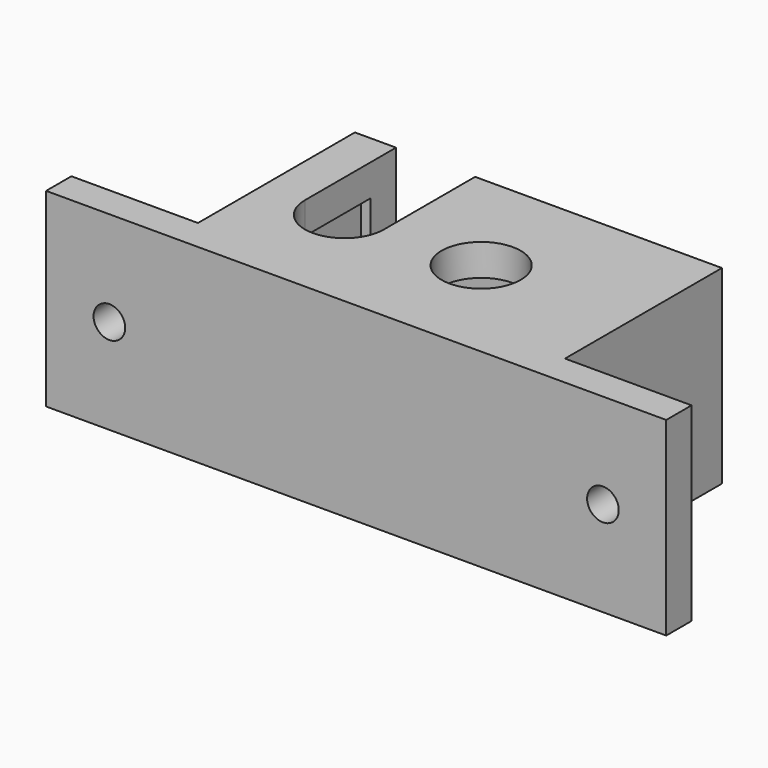
from build123d import *

# Parameters (mm, degrees)
F1_DEPTH = 30
F0_R     = 6.25
F2_DEPTH = 5
F3_W     = 5
F3_H     = 30
F4_DEPTH = 20
F5_W     = 5
F5_H     = 30
F6_DEPTH = 20
F7_R     = 2.5
F8_DEPTH = 25


# Not quite as in the source:
# - a feature names something its author has since deleted; it is built from what else it names


with BuildPart() as f1:
    # F0 (on Top) → F1 (new body)
    with BuildSketch(Plane.XY):
        Polygon((25.3224579843, 32.3690634753), (25.3224579843, 6.3690634753), (30.3224579843, 6.3690634753), (30.3224579843, 37.3690634753), (-8.6790506474, 37.3690634753), (-8.6790506474, 32.3690634753), align=None)
        Polygon((-22.6775420157, 6.3690634753), (-22.6775420157, 32.3690634753), (-21.1775420157, 32.3690634753), (-21.1775420157, 37.3690634753), (-27.6775420157, 37.3690634753), (-27.6775420157, 6.3690634753), align=None)
        Polygon((25.3224579843, 6.3690634753), (-22.6775420157, 6.3690634753), (-27.6775420157, 6.3690634753), (-27.6775420157, 1.3690634753), (30.3224579843, 1.3690634753), (30.3224579843, 6.3690634753), align=None)
    extrude(amount=-F1_DEPTH)

    # F0 (on Top) → F2 (join)
    with BuildSketch(Plane.XY):
        Polygon((-22.6775420157, 6.3690634753), (-22.6775420157, 32.3690634753), (-21.1775420157, 32.3690634753), (-21.1775420157, 37.3690634753), (-27.6775420157, 37.3690634753), (-27.6775420157, 6.3690634753), align=None)
        with BuildLine():
            Line((-21.1775420157, 32.3690634753), (-22.6775420157, 32.3690634753))
            Line((-22.6775420157, 32.3690634753), (-22.6775420157, 6.3690634753))
            Line((-22.6775420157, 6.3690634753), (25.3224579843, 6.3690634753))
            Line((25.3224579843, 6.3690634753), (25.3224579843, 32.3690634753))
            Line((25.3224579843, 32.3690634753), (-8.6790506474, 32.3690634753))
            Line((-8.6790506474, 32.3690634753), (-8.6790506474, 19.5063792474))
            ThreePointArc((-8.6790506474, 19.5063792474), (-14.858879986, 13.1194406446), (-21.1775420157, 19.3690634753))
            Line((-21.1775420157, 19.3690634753), (-21.1775420157, 32.3690634753))
        make_face()
        with Locations((6.6724579843, 19.3690634753)):
            Circle(F0_R, mode=Mode.SUBTRACT)
        Polygon((25.3224579843, 6.3690634753), (-22.6775420157, 6.3690634753), (-27.6775420157, 6.3690634753), (-27.6775420157, 1.3690634753), (30.3224579843, 1.3690634753), (30.3224579843, 6.3690634753), align=None)
        Polygon((25.3224579843, 32.3690634753), (25.3224579843, 6.3690634753), (30.3224579843, 6.3690634753), (30.3224579843, 37.3690634753), (-8.6790506474, 37.3690634753), (-8.6790506474, 32.3690634753), align=None)
    extrude(amount=-F2_DEPTH)

    # F3 (on face) → F4 (join)
    with BuildSketch(Plane.YZ.offset(30.3224579843)):
        with Locations((3.8690634753, -15)):
            Rectangle(F3_W, F3_H)
    extrude(amount=F4_DEPTH)

    # F5 (on face) → F6 (join)
    with BuildSketch(Plane(origin=(-27.6775420157, 0, 0), x_dir=(0, -1, 0), z_dir=(-1, 0, 0))):
        with Locations((-3.8690634753, -15)):
            Rectangle(F5_W, F5_H)
    extrude(amount=F6_DEPTH)

    # F7 (on face) → F8 (cut)
    with BuildSketch(Plane(origin=(0, 6.3690634753, 0), x_dir=(-1, 0, 0), z_dir=(0, 1, 0))):
        with Locations((-40.3224579843, -15)):
            Circle(F7_R)
        with Locations((37.6775420157, -15)):
            Circle(F7_R)
    extrude(amount=-F8_DEPTH, mode=Mode.SUBTRACT)


solid = f1.part
